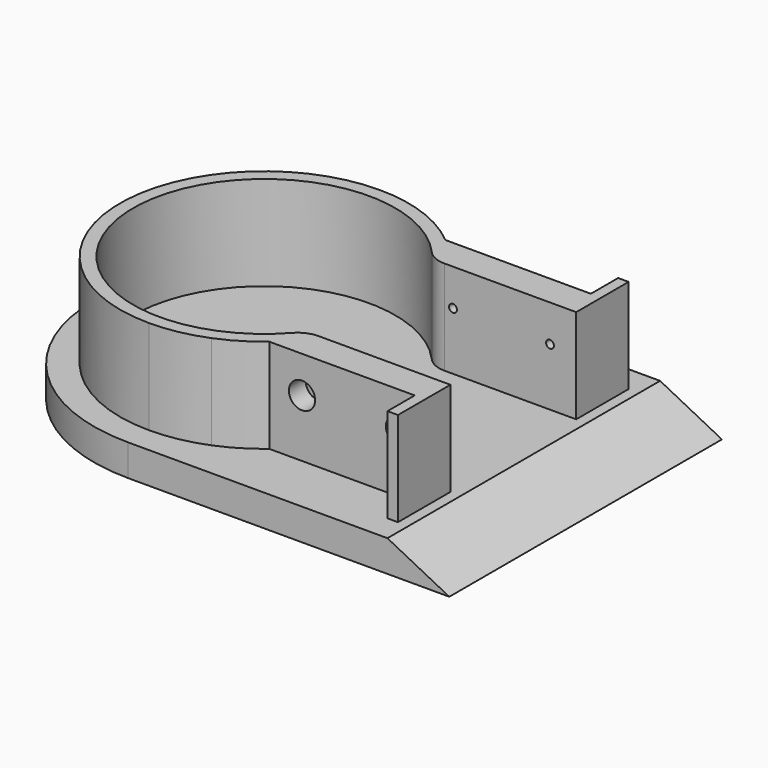
from build123d import *

# Parameters (mm, degrees)
F1_DEPTH = 24
F0_R     = 8.75
F2_DEPTH = 6
F4_DEPTH = 32.5
F5_R     = 5
F6_R     = 0.75
F7_DEPTH = 6
F6_R_2   = 2.5
F8_DEPTH = 4
F0_R_2   = 8
F9_DEPTH = 5


# Not quite as in the source:
# - a pattern or mirror of a feature is missing from the dataset's text; its kind, count and spacing are read off the source's solid


with BuildPart() as f1:
    # F0 (on Top) → F1 (new body)
    with BuildSketch(Plane.XY):
        with BuildLine():
            ThreePointArc((20, -15), (-25, 0), (20, 15))
            Line((20, 15), (47.5, 15))
            Line((47.5, 15), (47.5, 27.5))
            Line((47.5, 27.5), (45.5, 27.5))
            Line((45.5, 27.5), (45.5, 21))
            Line((45.5, 21), (39.5, 21))
            Line((39.5, 21), (28, 21))
            Line((28, 21), (17.7552809046, 21))
            ThreePointArc((17.7552809046, 21), (14.2047844975, 23.5472736719), (10.295630141, 25.5))
            ThreePointArc((10.295630141, 25.5), (5.2440442409, 26.9953699734), (0, 27.5))
            ThreePointArc((0, 27.5), (-27.5, 0), (0, -27.5))
            ThreePointArc((0, -27.5), (5.2440442409, -26.9953699734), (10.295630141, -25.5))
            ThreePointArc((10.295630141, -25.5), (14.2047844975, -23.5472736719), (17.7552809046, -21))
            Line((17.7552809046, -21), (28, -21))
            Line((28, -21), (39.5, -21))
            Line((39.5, -21), (45.5, -21))
            Line((45.5, -21), (45.5, -27.5))
            Line((45.5, -27.5), (47.5, -27.5))
            Line((47.5, -27.5), (47.5, -15))
            Line((47.5, -15), (20, -15))
        make_face()
    extrude(amount=F1_DEPTH)

    # F0 (on Top) → F2 (join)
    with BuildSketch(Plane.XY):
        with BuildLine():
            Line((47.5, 15), (20, 15))
            ThreePointArc((20, 15), (-25, 0), (20, -15))
            Line((20, -15), (47.5, -15))
            Line((47.5, -15), (47.5, 15))
        make_face()
        Circle(F0_R, mode=Mode.SUBTRACT)
        with BuildLine():
            Line((45.5, 21), (45.5, 27.5))
            Line((45.5, 27.5), (0, 27.5))
            ThreePointArc((0, 27.5), (5.2440442409, 26.9953699734), (10.295630141, 25.5))
            ThreePointArc((10.295630141, 25.5), (14.2047844975, 23.5472736719), (17.7552809046, 21))
            Line((17.7552809046, 21), (28, 21))
            Line((28, 21), (39.5, 21))
            Line((39.5, 21), (45.5, 21))
        make_face()
        with BuildLine():
            Line((0, -27.5), (45.5, -27.5))
            Line((45.5, -27.5), (45.5, -21))
            Line((45.5, -21), (39.5, -21))
            Line((39.5, -21), (28, -21))
            Line((28, -21), (17.7552809046, -21))
            ThreePointArc((17.7552809046, -21), (14.2047844975, -23.5472736719), (10.295630141, -25.5))
            ThreePointArc((10.295630141, -25.5), (5.2440442409, -26.9953699734), (0, -27.5))
        make_face()
        Polygon((47.5, 27.5), (47.5, 15), (47.5, -15), (47.5, -27.5), (49.5, -27.5), (49.5, 27.5), align=None)
        with BuildLine():
            Line((45.5, 27.5), (47.5, 27.5))
            Line((47.5, 27.5), (49.5, 27.5))
            Line((49.5, 27.5), (49.5, 32.5))
            Line((49.5, 32.5), (0, 32.5))
            ThreePointArc((0, 32.5), (-32.5, 0), (0, -32.5))
            Line((0, -32.5), (49.5, -32.5))
            Line((49.5, -32.5), (49.5, -27.5))
            Line((49.5, -27.5), (47.5, -27.5))
            Line((47.5, -27.5), (45.5, -27.5))
            Line((45.5, -27.5), (0, -27.5))
            ThreePointArc((0, -27.5), (-27.5, 0), (0, 27.5))
            Line((0, 27.5), (45.5, 27.5))
        make_face()
    extrude(amount=F2_DEPTH)

    # F3 (on Front) → F4 (join, symmetric)
    with BuildSketch(Plane.XZ):
        Polygon((49.5, 6), (49.5, 0), (61.2984150648, 0), align=None)
    extrude(amount=F4_DEPTH, both=True)

    # F5
    f5_edges = [f1.edges().sort_by_distance(p)[0] for p in [
        (20, 15, 15),
        (20, -15, 15),
    ]]
    fillet(f5_edges, radius=F5_R)

    # F6 (on face) → F7 (cut, through all)
    with BuildSketch(Plane.XZ.offset(21)):
        with Locations((24, 17)):
            Circle(F6_R)
        with Locations((42.5, 17)):
            Circle(F6_R)
    f7 = extrude(amount=-F7_DEPTH, mode=Mode.SUBTRACT)

    # F7_copies: F7 across plane
    add(f7.mirror(Plane.ZX), mode=Mode.SUBTRACT)

    # F6 (on face) → F8 (cut)
    with BuildSketch(Plane.XZ.offset(21)):
        with Locations((24, 17)):
            Circle(F6_R_2)
        with Locations((24, 17)):
            Circle(F6_R, mode=Mode.SUBTRACT)
        with Locations((42.5, 17)):
            Circle(F6_R_2)
        with Locations((42.5, 17)):
            Circle(F6_R, mode=Mode.SUBTRACT)
    f8 = extrude(amount=-F8_DEPTH, mode=Mode.SUBTRACT)

    # F8_copies: F8 across plane
    add(f8.mirror(Plane.ZX), mode=Mode.SUBTRACT)

    # F0 (on Top) → F9 (join)
    with BuildSketch(Plane.XY):
        Circle(F0_R)
        Circle(F0_R_2, mode=Mode.SUBTRACT)
    extrude(amount=F9_DEPTH)


solid = f1.part
